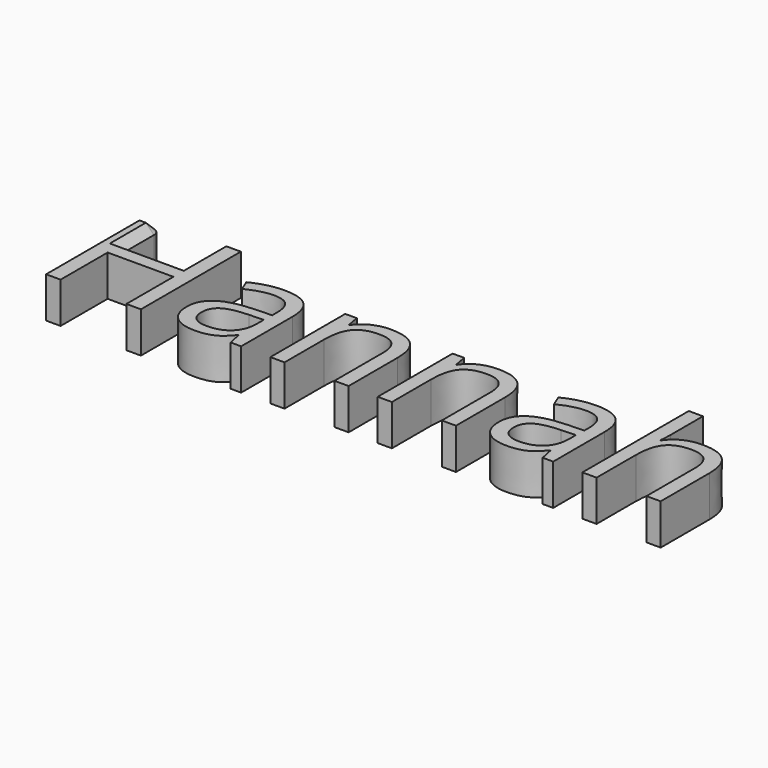
from build123d import *

# Parameters (mm, degrees)
F0_TEXT_SIZE = 107.2524606975
F1_DEPTH     = 25
F2_R         = 5
F3_T1_DEPTH  = 27.5779349369
F3_T3_DEPTH  = 16.7570175383
F3_T6_ANGLE  = 90


# Not quite as in the source:
# - a fillet or chamfer that OpenCascade refuses, or shapes differently, is made with other operations: its cross-section is extruded or revolved along the edge and cut away or added
# - Text() gives the source's letters only with a copy of the font that has no kerning and outlines rounded to 1/6400 em; it was checked with that copy


with BuildPart() as f1:
    # F0 (on Top) → F1 (new body)
    with BuildSketch(Plane.XY):
        with Locations((-394.2198258511, -60.5236366391)):
            Text('Hannah', F0_TEXT_SIZE, font='Open Sans', text_align=(TextAlign.LEFT, TextAlign.BOTTOM))
    extrude(amount=F1_DEPTH)

    # F2
    f2_edges = [f1.edges().sort_by_distance(p)[0] for p in [
        (-374.797076, 16.044565, 12.5),
    ]]
    fillet(f2_edges, radius=F2_R)

    # F3: chamfer of 5 on 3 edges, made by hand

    # F3_s2 → F3_t1 (cut)
    with BuildSketch(Plane.XZ.offset(-11.0445653807)):
        Polygon((-374.7970755467, 20), (-379.7970755467, 25), (-374.7970755467, 25), align=None)
    extrude(amount=F3_T1_DEPTH, mode=Mode.SUBTRACT)

    # F3_s4 → F3_t3 (cut)
    with BuildSketch(Plane.YZ.offset(-396.554093085)):
        Polygon((11.0445653807, 25), (16.0445653807, 20), (16.0445653807, 25), align=None)
    extrude(amount=F3_T3_DEPTH, mode=Mode.SUBTRACT)

    # F3_s5 → F3_t6 (revolve, cut)
    with BuildSketch(Plane.XZ.offset(-11.0445653807)):
        Polygon((-374.7970755467, 20), (-379.7970755467, 25), (-374.7970755467, 25), align=None)
    revolve(axis=Axis((-379.7970755467, 11.0445653807, 25), (0, 0, 1)), revolution_arc=F3_T6_ANGLE, mode=Mode.SUBTRACT)


solid = f1.part
